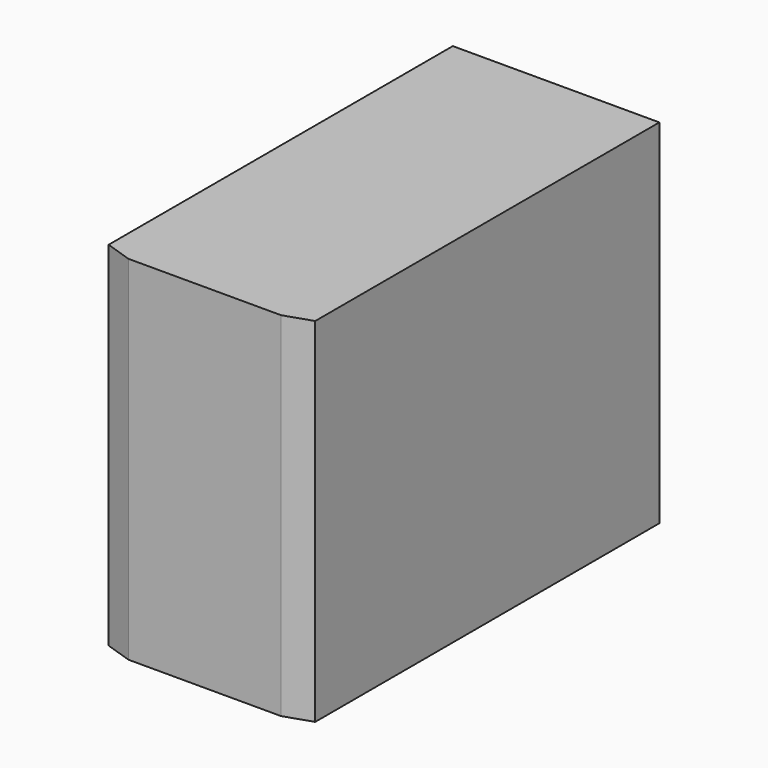
from build123d import *

# Parameters (mm, degrees)
F0_W     = 230
F0_H     = 393
F1_DEPTH = 489
F2_SIZE2 = 10
F2_SIZE  = 30


with BuildPart() as f1:
    # F0 (on Front) → F1 (new body)
    with BuildSketch(Plane.XZ):
        with Locations((115, 196.5)):
            Rectangle(F0_W, F0_H)
    extrude(amount=-F1_DEPTH)

    # F2
    f2_edges = [f1.edges().sort_by_distance(p)[0] for p in [
        (230, 0, 196.5),
        (0, 0, 196.5),
    ]]
    f2_side = f1.faces().sort_by_distance((115, 0, 196.5))[0]
    chamfer(f2_edges, length=F2_SIZE, length2=F2_SIZE2, reference=f2_side)


solid = f1.part
